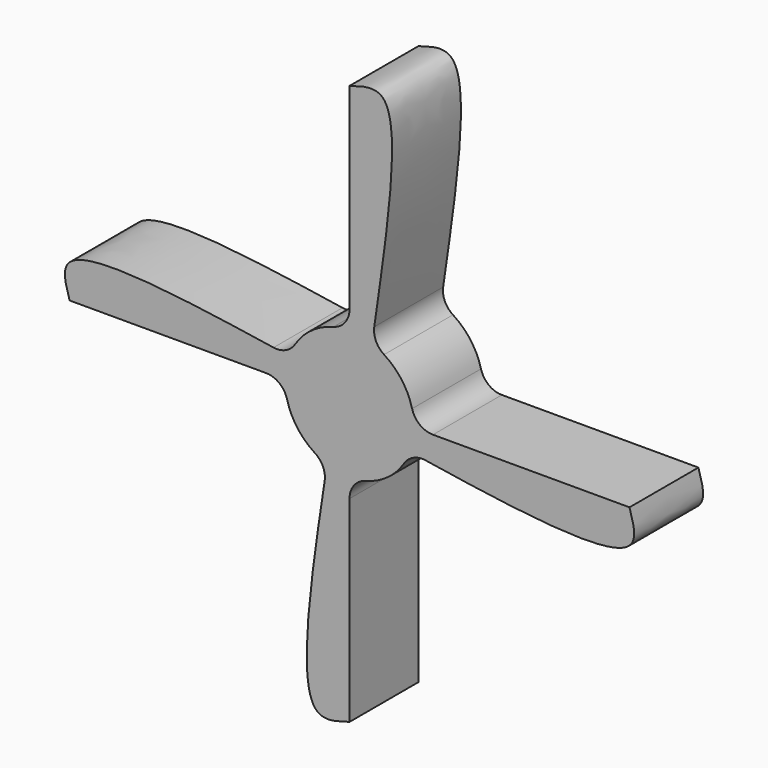
from build123d import *

# Parameters (mm, degrees)
F0_R     = 15
F1_DEPTH = 20
F3_DEPTH = 20
F4_R     = 5


with BuildPart() as f1:
    # F0 (on Front) → F1 (new body)
    with BuildSketch(Plane.XZ):
        Circle(F0_R)
    extrude(amount=F1_DEPTH)

    # F2 (on face) → F3 (join)
    with BuildSketch(Plane.XZ.offset(20)):
        with BuildLine():
            ThreePointArc((-15, 0), (-14.7631627709, 2.655), (-14.06013, 5.2261596209))
            add(Edge.make_bspline(
                [(-65, 0), (-65.9329413789, 3.010937683), (-69.2521733617, 13.7232941953), (-37.1437743961, 8.7800203036), (-14.06013, 5.2261596209)],
                knots=[0, 0, 0, 0, 0.2810714598, 1, 1, 1, 1], degree=3))
            Line((-65, 0), (-15, 0))
        make_face()
        with BuildLine():
            Line((0, 65), (0, 15))
            ThreePointArc((0, 15), (2.655, 14.7631627709), (5.2261596209, 14.06013))
            add(Edge.make_bspline(
                [(0, 65), (3.004974431, 65.9351556825), (13.7758270003, 69.2317905803), (8.5502960631, 37.2335582385), (5.2261596209, 14.06013)],
                knots=[0, 0, 0, 0, 0.2810714598, 1, 1, 1, 1], degree=3))
        make_face()
        with BuildLine():
            Line((65, 0), (15, 0))
            ThreePointArc((15, 0), (14.7631627709, -2.655), (14.06013, -5.2261596209))
            add(Edge.make_bspline(
                [(65, 0), (65.9317768654, -3.0153578506), (69.2624940597, -13.6887766969), (37.0985962701, -8.9276804293), (14.06013, -5.2261596209)],
                knots=[0, 0, 0, 0, 0.2810714598, 1, 1, 1, 1], degree=3))
        make_face()
        with BuildLine():
            ThreePointArc((0, -15), (-2.655, -14.7631627709), (-5.2261596209, -14.06013))
            add(Edge.make_bspline(
                [(0, -65), (-3.0107097333, -65.9328713139), (-13.7231855798, -69.252502796), (-8.7790973132, -37.1419421153), (-5.2261596209, -14.06013)],
                knots=[0, 0, 0, 0, 0.2810678576, 1, 1, 1, 1], degree=3))
            Line((0, -65), (0, -15))
        make_face()
    extrude(amount=-F3_DEPTH)

    # F4
    f4_edges = [f1.edges().sort_by_distance(p)[0] for p in [
        (15, -10, 0),
        (5.22616, -10, 14.06013),
        (-14.06013, -10, 5.22616),
        (0, -10, 15),
        (-5.22616, -10, -14.06013),
        (-15, -10, 0),
        (14.06013, -10, -5.22616),
        (0, -10, -15),
    ]]
    fillet(f4_edges, radius=F4_R)


solid = f1.part
